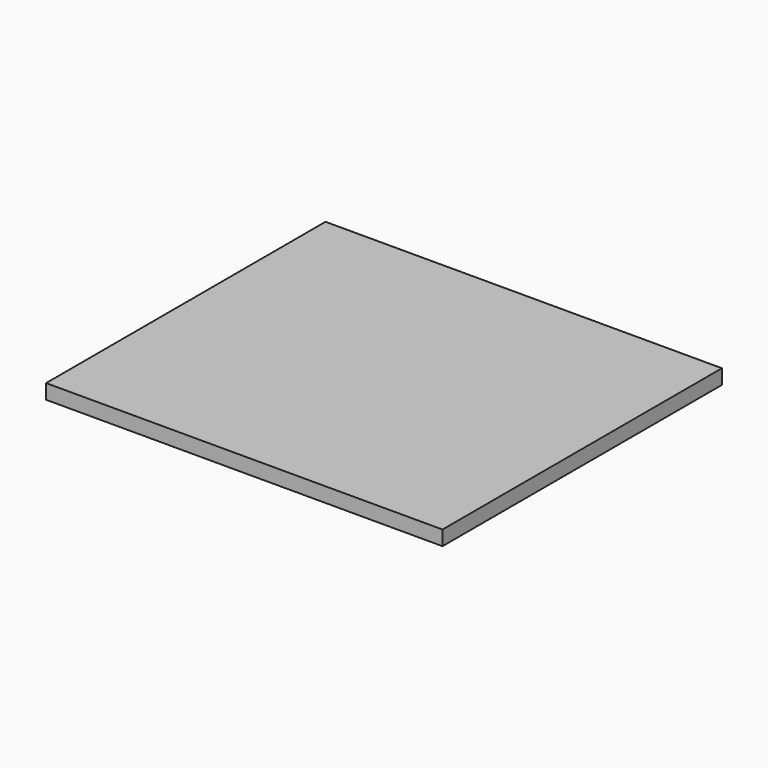
from build123d import *

# Parameters (mm, degrees)
F0_W     = 136.9314
F0_H     = 120.65
F2_DEPTH = 5.08
F1_W     = 85.725
F1_H     = 55.5625
F1_W_2   = 68.58
F1_H_2   = 53.34
F1_R     = 1.5875
F3_DEPTH = 3.175


# Not quite as in the source:
# - the program builds the solid bodies; features that only make, move or delete a surface that nothing else refers to are left out


with BuildPart() as f2:
    # F0 (on Top) → F2 (new body)
    with BuildSketch(Plane.XY):
        Rectangle(F0_W, F0_H)
    extrude(amount=F2_DEPTH)

    # F1 (on Top) → F3 (cut)
    with BuildSketch(Plane.XY):
        with Locations((17.2909619287, 28.73375)):
            Rectangle(F1_W, F1_H)
        with Locations((25.8121827105, -29.845)):
            Rectangle(F1_W_2, F1_H_2)
        with Locations((5.4921827105, -53.975)):
            Circle(F1_R, mode=Mode.SUBTRACT)
        with Locations((6.7621827105, -5.715)):
            Circle(F1_R, mode=Mode.SUBTRACT)
        with Locations((57.5621827105, -48.895)):
            Circle(F1_R, mode=Mode.SUBTRACT)
        with Locations((57.5621827105, -20.955)):
            Circle(F1_R, mode=Mode.SUBTRACT)
    extrude(amount=F3_DEPTH, mode=Mode.SUBTRACT)


solid = f2.part
